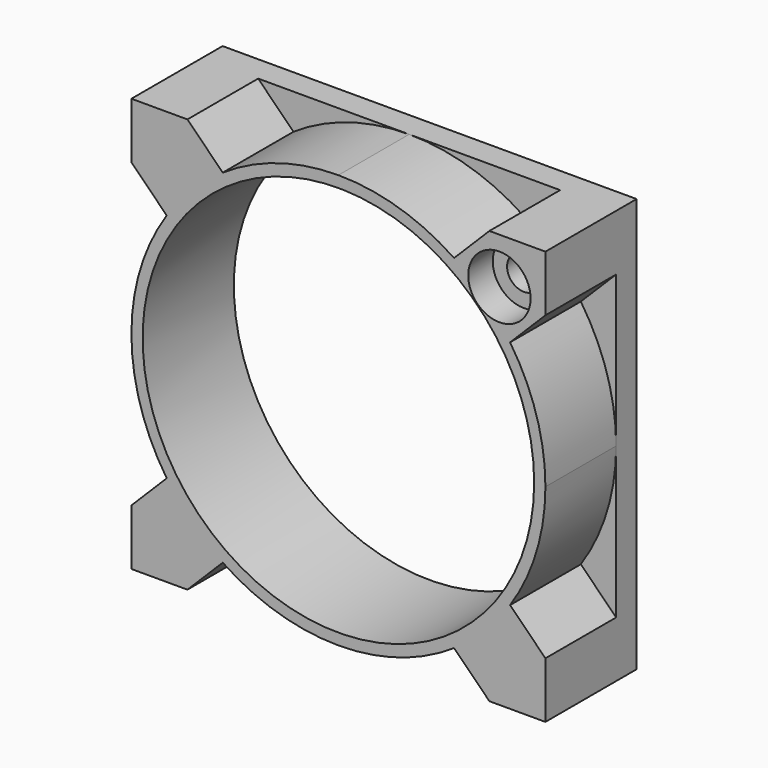
from build123d import *

# Parameters (mm, degrees)
F0_W            = 40.5
F0_H            = 40.5
F1_DEPTH        = 2.5
F3_DEPTH        = 8.65
F4_DEPTH        = 8.65
F4_COPIES_COUNT = 4
F5_R            = 19.15
F6_DEPTH        = 11.151
F8_D            = 3.3
F8_CBORE_D      = 6.1
F8_CBORE_DEPTH  = 3


# Not quite as in the source:
# - a pattern or mirror of a feature is missing from the dataset's text; its kind, count and spacing are read off the source's solid


with BuildPart() as f1:
    # F0 (on Front) → F1 (new body)
    with BuildSketch(Plane.XZ):
        with Locations((20.25, 20.25)):
            Rectangle(F0_W, F0_H)
    extrude(amount=F1_DEPTH)

    # F2 (on face) → F3 (join)
    with BuildSketch(Plane.XZ.offset(2.5)):
        with BuildLine():
            ThreePointArc((20.25, 0), (34.568912319, 5.931087681), (40.5, 20.25))
            ThreePointArc((40.5, 20.25), (39.6168263322, 26.1651109727), (37.0443419437, 31.5642643895))
            ThreePointArc((37.0443419437, 31.5642643895), (34.568912319, 34.568912319), (31.5642643895, 37.0443419437))
            ThreePointArc((31.5642643895, 37.0443419437), (26.1651109727, 39.6168263322), (20.25, 40.5))
            ThreePointArc((20.25, 40.5), (5.931087681, 34.568912319), (0, 20.25))
            ThreePointArc((0, 20.25), (5.931087681, 5.931087681), (20.25, 0))
        make_face()
    extrude(amount=F3_DEPTH)

    # F2 (on face) → F4 (join, through all)
    with BuildSketch(Plane.XZ.offset(2.5)):
        with BuildLine():
            ThreePointArc((31.5642643895, 37.0443419437), (34.568912319, 34.568912319), (37.0443419437, 31.5642643895))
            Line((37.0443419437, 31.5642643895), (40.5, 35.0199224458))
            Line((40.5, 35.0199224458), (40.5, 40.5))
            Line((40.5, 40.5), (35.0199224458, 40.5))
            Line((35.0199224458, 40.5), (31.5642643895, 37.0443419437))
        make_face()
    f4 = extrude(amount=F4_DEPTH)

    # F4_copies: F4 ×4 about axis
    f4_copies_axis = Axis((20.25, 0, 20.25), (0, 1, 0))
    for i in range(1, F4_COPIES_COUNT):
        add(f4.rotate(f4_copies_axis, i * 360 / F4_COPIES_COUNT))

    # F5 (on face) → F6 (cut, through all)
    with BuildSketch(Plane.XZ.offset(11.15)):
        with Locations((20.25, 20.25)):
            Circle(F5_R)
    extrude(amount=-F6_DEPTH, mode=Mode.SUBTRACT)

    # F8 (through all)
    with Locations(Plane.XZ.offset(11.15)):
        with Locations((36, 36)):
            CounterBoreHole(F8_D / 2, F8_CBORE_D / 2, F8_CBORE_DEPTH)


solid = f1.part
